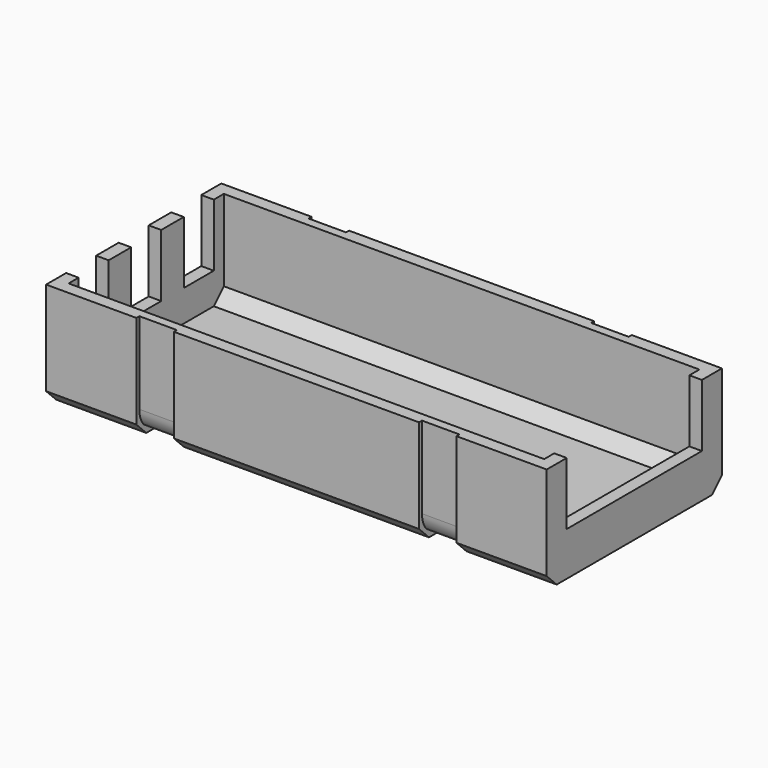
from build123d import *

# Parameters (mm, degrees)
F0_W         = 40
F0_H         = 17.5
F1_DEPTH     = 8.5
F2_T         = -1
F3_W         = 1
F3_H         = 3
F4_DEPTH     = 5
F5_SIZE      = 1
F8_W         = 3
F8_H         = 1
F8_H_2       = 7.5
F11_DEPTH    = 0.3
F7_W         = 3
F7_H         = 1.4142135624
F12_DEPTH    = 0.3
F6_W         = 3
F6_H         = 15.5
F13_DEPTH    = 0.3
F9_W         = 3
F9_H         = 7.5
F14_DEPTH    = 0.3
F10_W        = 3
F10_H        = 5.3033008589
F10_H_2      = 1.4142135624
F15_DEPTH    = 0.3
F16_T1_DEPTH = 3
F16_T3_DEPTH = 3
F18_W        = 2.25
F18_H        = 5
F19_DEPTH    = 25


# Not quite as in the source:
# - a fillet or chamfer that OpenCascade refuses, or shapes differently, is made with other operations: its cross-section is extruded or revolved along the edge and cut away or added
# - two fillets or chamfers of one size are made in one step


with BuildPart() as f1:
    # F0 (on Top) → F1 (new body)
    with BuildSketch(Plane.XY):
        with Locations((-65.668810606, 16.5984117985)):
            Rectangle(F0_W, F0_H)
    extrude(amount=F1_DEPTH)

    # F2
    f2_openings = [f1.faces().sort_by_distance(p)[0] for p in [
        (-65.668811, 16.598412, 8.5),
    ]]
    offset(amount=F2_T, openings=f2_openings)

    # F3 (on face) → F4 (cut)
    with BuildSketch(Plane.XY.offset(8.5)):
        with Locations((-85.168810606, 21.8484117985)):
            Rectangle(F3_W, F3_H)
        with Locations((-85.168810606, 16.5984117985)):
            Rectangle(F3_W, F3_H)
        with Locations((-85.168810606, 11.3484117985)):
            Rectangle(F3_W, F3_H)
        with Locations((-46.168810606, 11.3484117985)):
            Rectangle(F3_W, F3_H)
        with Locations((-46.168810606, 16.5984117985)):
            Rectangle(F3_W, F3_H)
        with Locations((-46.168810606, 21.8484117985)):
            Rectangle(F3_W, F3_H)
    extrude(amount=-F4_DEPTH, mode=Mode.SUBTRACT)

    # F5
    f5_edges = [f1.edges().sort_by_distance(p)[0] for p in [
        (-65.668811, 7.848412, 0),
        (-65.668811, 25.348412, 0),
        (-65.668811, 24.348412, 1),
        (-65.668811, 8.848412, 1),
    ]]
    chamfer(f5_edges, length=F5_SIZE)

    # F8 (on face) → F11 (cut)
    with BuildSketch(Plane(origin=(0, 25.3484117985, 0), x_dir=(-1, 0, 0), z_dir=(0, 1, 0))):
        with Locations((76.9616991878, 0.5)):
            Rectangle(F8_W, F8_H)
        with Locations((76.9616991878, 4.75)):
            Rectangle(F8_W, F8_H_2)
        with Locations((54.3759220243, 4.75)):
            Rectangle(F8_W, F8_H_2)
    extrude(amount=-F11_DEPTH, mode=Mode.SUBTRACT)

    # F7 (on face) → F12 (cut)
    with BuildSketch(Plane(origin=(0, 12.1742058992, -12.1742058992), x_dir=(1, 0, 0), z_dir=(0, 0.7071067812, -0.7071067812))):
        with Locations((-76.9616991878, -17.924033875)):
            Rectangle(F7_W, F7_H)
        with Locations((-54.3759220243, -17.924033875)):
            Rectangle(F7_W, F7_H)
    extrude(amount=-F12_DEPTH, mode=Mode.SUBTRACT)

    # F6 (on face) → F13 (cut)
    with BuildSketch(Plane(origin=(0, 0, 0), x_dir=(1, 0, 0), z_dir=(0, 0, -1))):
        with Locations((-76.9616991878, -16.5984117985)):
            Rectangle(F6_W, F6_H)
        with Locations((-54.3759220243, -16.5984117985)):
            Rectangle(F6_W, F6_H)
    extrude(amount=-F13_DEPTH, mode=Mode.SUBTRACT)

    # F9 (on face) → F14 (cut)
    with BuildSketch(Plane.XZ.offset(-7.8484117985)):
        with Locations((-76.9616991878, 4.75)):
            Rectangle(F9_W, F9_H)
        with Locations((-54.3759220243, 4.75)):
            Rectangle(F9_W, F9_H)
    extrude(amount=-F14_DEPTH, mode=Mode.SUBTRACT)

    # F10 (on face) → F15 (cut)
    with BuildSketch(Plane(origin=(0, 4.4242058992, 4.4242058992), x_dir=(1, 0, 0), z_dir=(0, -0.7071067812, -0.7071067812))):
        with Locations((-76.9616991878, -2.1909079936)):
            Rectangle(F10_W, F10_H)
        with Locations((-76.9616991878, -5.5496652042)):
            Rectangle(F10_W, F10_H_2)
        with Locations((-54.3759220243, -5.5496652042)):
            Rectangle(F10_W, F10_H_2)
    extrude(amount=-F15_DEPTH, mode=Mode.SUBTRACT)

    # F16: fillet of radius 2 on 8 edges, made by hand

    # F16_s2 → F16_t1 (cut)
    with BuildSketch(Plane.YZ.offset(-55.8759220243)):
        with BuildLine():
            ThreePointArc((8.7341982361, 0.5384776311), (8.3006527335, 1.1873243287), (8.1484117985, 1.9526911935))
            Line((8.1484117985, 1.9526911935), (8.1484117985, 1.1242640687))
            Line((8.1484117985, 1.1242640687), (8.7341982361, 0.5384776311))
        make_face()
        with BuildLine():
            ThreePointArc((9.8011029919, 0.3), (9.0357361272, 0.452240935), (8.3868894296, 0.8857864376))
            Line((8.3868894296, 0.8857864376), (8.9726758672, 0.3))
            Line((8.9726758672, 0.3), (9.8011029919, 0.3))
        make_face()
        with BuildLine():
            ThreePointArc((25.0484117985, 1.9526911935), (24.8961708635, 1.1873243287), (24.4626253609, 0.5384776311))
            Line((24.4626253609, 0.5384776311), (25.0484117985, 1.1242640687))
            Line((25.0484117985, 1.1242640687), (25.0484117985, 1.9526911935))
        make_face()
        with BuildLine():
            ThreePointArc((24.8099341674, 0.8857864376), (24.1610874697, 0.452240935), (23.395720605, 0.3))
            Line((23.395720605, 0.3), (24.2241477298, 0.3))
            Line((24.2241477298, 0.3), (24.8099341674, 0.8857864376))
        make_face()
    extrude(amount=F16_T1_DEPTH, mode=Mode.SUBTRACT)

    # F16_s4 → F16_t3 (cut)
    with BuildSketch(Plane.YZ.offset(-78.4616991878)):
        with BuildLine():
            ThreePointArc((9.8011029919, 0.3), (9.0357361272, 0.452240935), (8.3868894296, 0.8857864376))
            Line((8.3868894296, 0.8857864376), (8.9726758672, 0.3))
            Line((8.9726758672, 0.3), (9.8011029919, 0.3))
        make_face()
        with BuildLine():
            ThreePointArc((8.7341982361, 0.5384776311), (8.3006527335, 1.1873243287), (8.1484117985, 1.9526911935))
            Line((8.1484117985, 1.9526911935), (8.1484117985, 1.1242640687))
            Line((8.1484117985, 1.1242640687), (8.7341982361, 0.5384776311))
        make_face()
        with BuildLine():
            ThreePointArc((24.8099341674, 0.8857864376), (24.1610874697, 0.452240935), (23.395720605, 0.3))
            Line((23.395720605, 0.3), (24.2241477298, 0.3))
            Line((24.2241477298, 0.3), (24.8099341674, 0.8857864376))
        make_face()
        with BuildLine():
            ThreePointArc((25.0484117985, 1.9526911935), (24.8961708635, 1.1873243287), (24.4626253609, 0.5384776311))
            Line((24.4626253609, 0.5384776311), (25.0484117985, 1.1242640687))
            Line((25.0484117985, 1.1242640687), (25.0484117985, 1.9526911935))
        make_face()
    extrude(amount=F16_T3_DEPTH, mode=Mode.SUBTRACT)

    # F18 (on face) → F19 (cut)
    with BuildSketch(Plane.YZ.offset(-45.668810606)):
        with Locations((13.9734117985, 6)):
            Rectangle(F18_W, F18_H)
        with Locations((19.2234117985, 6)):
            Rectangle(F18_W, F18_H)
    extrude(amount=-F19_DEPTH, mode=Mode.SUBTRACT)


solid = f1.part
